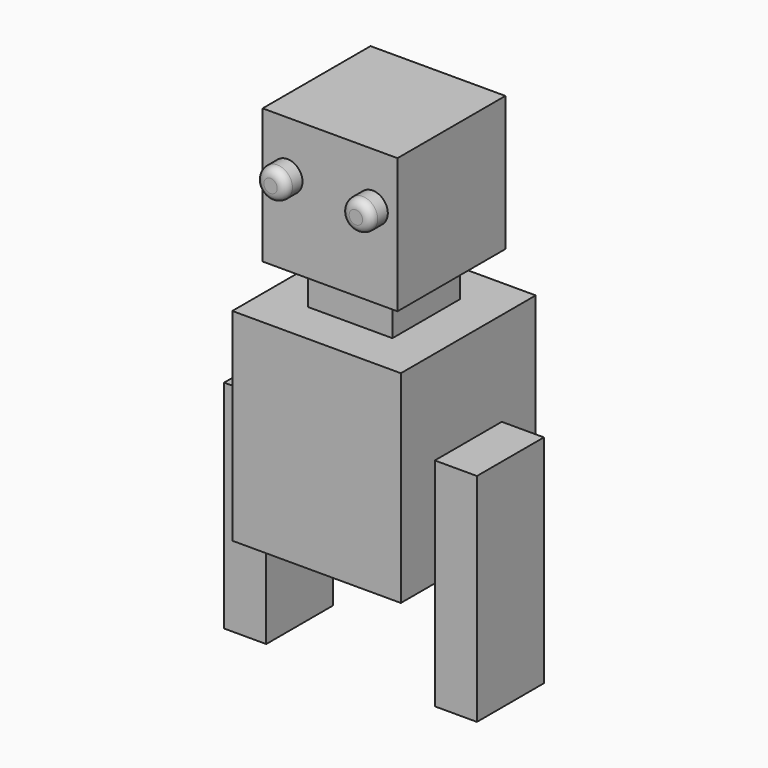
from build123d import *

# Parameters (mm, degrees)
F0_W      = 100
F0_H      = 100
F1_DEPTH  = 120
F2_W      = 50
F2_H      = 50
F3_DEPTH  = 50
F5_W      = 80
F5_H      = 80
F6_DEPTH  = 80
F9_DEPTH  = 10
F10_W     = 49.6545396745
F10_H     = 64.2159506679
F11_DEPTH = 25
F15_R     = 8.949511536
F16_DEPTH = 12.5
F19_R     = 5
F19_2_R   = 5


with BuildPart() as f1:
    # F0 (on Top) → F1 (new body)
    with BuildSketch(Plane.XY):
        Rectangle(F0_W, F0_H)
    extrude(amount=F1_DEPTH)

    # F2 (on face) → F3 (join)
    with BuildSketch(Plane.XY.offset(120)):
        Rectangle(F2_W, F2_H)
    extrude(amount=F3_DEPTH)


with BuildPart() as f6:
    # F5 (on offset) → F6 (new body)
    with BuildSketch(Plane.XY.offset(145)):
        Rectangle(F5_W, F5_H)
    extrude(amount=F6_DEPTH)

    # F7: cut F1
    add(f1.part, mode=Mode.SUBTRACT)


with BuildPart() as f9:
    # F8 (on face) → F9 (new body)
    with BuildSketch(Plane.YZ.offset(50)):
        with BuildLine():
            ThreePointArc((10, 40), (-7.0710678119, 47.0710678119), (0, 30))
            ThreePointArc((0, 30), (7.0710678119, 32.9289321881), (10, 40))
        make_face()
    extrude(amount=-F9_DEPTH)

    # F10 (on face) → F11 (join)
    with BuildSketch(Plane.YZ.offset(50)):
        with Locations((0, 32.1079753339)):
            Rectangle(F10_W, F10_H)
        with Locations((0, -32.1079753339)):
            Rectangle(F10_W, F10_H)
    extrude(amount=F11_DEPTH)


with BuildPart() as f1_1:
    add(f1.part)

    # F12: cut F9
    add(f9.part, mode=Mode.SUBTRACT)


with BuildPart() as f13_1:
    # F13: instance of F9
    add(f9.part.mirror(Plane.YZ))


with BuildPart() as f1_2:
    add(f1_1.part)

    # F14: cut F13_1
    add(f13_1.part, mode=Mode.SUBTRACT)


with BuildPart() as f16:
    # F15 (on face) → F16 (new body, symmetric)
    with BuildSketch(Plane.XZ.offset(40)):
        with Locations((-25.2957064658, 194.3687796593)):
            Circle(F15_R)
    extrude(amount=F16_DEPTH, both=True)


with BuildPart() as f17_1:
    # F17: instance of F16
    add(f16.part.mirror(Plane.YZ))


with BuildPart() as f6_1:
    add(f6.part)

    # F18: cut F16, F17_1
    add(f16.part, mode=Mode.SUBTRACT)
    add(f17_1.part, mode=Mode.SUBTRACT)


with BuildPart() as f16_1:
    add(f16.part)

    # F19
    f19_edges = [f16_1.edges().sort_by_distance(p)[0] for p in [
        (-34.245218, -52.5, 194.36878),
    ]]
    fillet(f19_edges, radius=F19_R)


with BuildPart() as f17_1_1:
    add(f17_1.part)

    # F19#2
    f19_2_edges = [f17_1_1.edges().sort_by_distance(p)[0] for p in [
        (34.245218, -52.5, 194.36878),
    ]]
    fillet(f19_2_edges, radius=F19_2_R)


solid = Compound([f9.part, f13_1.part, f1_2.part, f6_1.part, f16_1.part, f17_1_1.part])
